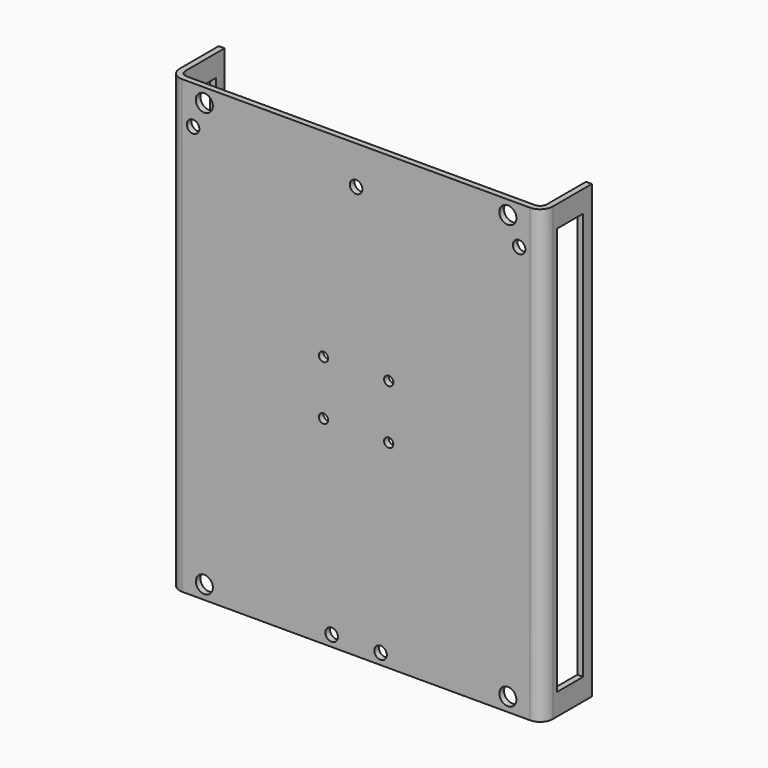
from build123d import *

# Parameters (mm, degrees)
F1_DEPTH  = 131.8250094
F2_W      = 9.525
F2_H      = 119.1250094
F3_DEPTH  = 108.98632
F4_R      = 3.69316
F5_R      = 1.98374
F6_R      = 1.8288
F7_DEPTH  = 257
F8_R      = 2.5
F9_DEPTH  = 1.70942
F10_R     = 1.35255
F11_DEPTH = 1.70942


# Not quite as in the source:
# - an extrude ends at something that could not be found from the text; its depth is read off the source's solid


with BuildPart() as f1:
    # F0 (on Top) → F1 (new body)
    with BuildSketch(Plane.XY):
        Polygon((0, 16.27124), (0, 0), (-105.56748, 0), (-105.56748, 16.27124), (-107.2769, 16.27124), (-107.2769, -1.70942), (1.70942, -1.70942), (1.70942, 16.27124), align=None)
    extrude(amount=F1_DEPTH)

    # F2 (on face) → F3 (cut, through all)
    with BuildSketch(Plane.YZ.offset(1.70942)):
        with Locations((8.33374, 65.9125047)):
            Rectangle(F2_W, F2_H)
    extrude(amount=-F3_DEPTH, mode=Mode.SUBTRACT)

    # F4
    f4_edges = [f1.edges().sort_by_distance(p)[0] for p in [
        (1.70942, -1.70942, 65.912505),
        (-107.2769, -1.70942, 65.912505),
    ]]
    fillet(f4_edges, radius=F4_R)

    # F5
    f5_edges = [f1.edges().sort_by_distance(p)[0] for p in [
        (0, 0, 65.912505),
        (-105.56748, 0, 65.912505),
    ]]
    fillet(f5_edges, radius=F5_R)

    # F6 (on face) → F7 (cut, through all)
    with BuildSketch(Plane.XZ.offset(1.70942)):
        with Locations((-52.78374, 120.65)):
            Circle(F6_R)
        with Locations((-5.15874, 120.65)):
            Circle(F6_R)
        with Locations((-100.40874, 120.65)):
            Circle(F6_R)
        with Locations((-45.63999, 3.175)):
            Circle(F6_R)
        with Locations((-59.92749, 3.175)):
            Circle(F6_R)
    extrude(amount=-F7_DEPTH, mode=Mode.SUBTRACT)

    # F8 (on face) → F9 (cut, through all)
    with BuildSketch(Plane.XZ.offset(1.70942)):
        with Locations((-8.452485, 127.8250094)):
            Circle(F8_R)
        with Locations((-8.452485, 4)):
            Circle(F8_R)
        with Locations((-97.114995, 4)):
            Circle(F8_R)
        with Locations((-97.114995, 127.8250094)):
            Circle(F8_R)
    extrude(amount=-F9_DEPTH, mode=Mode.SUBTRACT)

    # F10 (on face) → F11 (cut, through all)
    with BuildSketch(Plane.XZ.offset(1.70942)):
        with Locations((-43.25874, 57.9750047)):
            Circle(F10_R)
        with Locations((-43.25874, 73.8500047)):
            Circle(F10_R)
        with Locations((-62.30874, 57.9750047)):
            Circle(F10_R)
        with Locations((-62.30874, 73.8500047)):
            Circle(F10_R)
    extrude(amount=-F11_DEPTH, mode=Mode.SUBTRACT)


solid = f1.part
